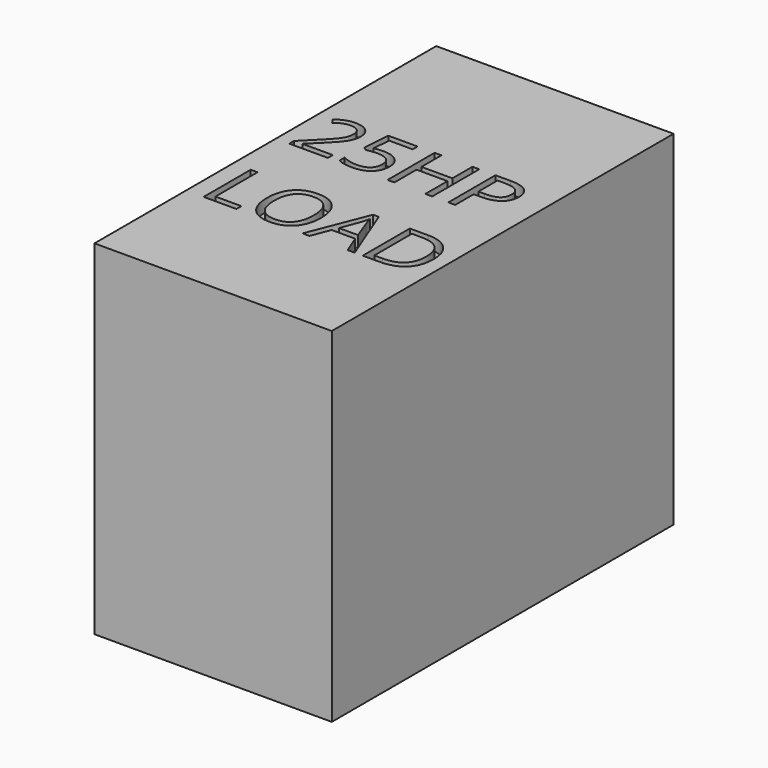
from build123d import *

# Parameters (mm, degrees)
F0_W         = 101.6
F0_H         = 182.88
F1_DEPTH     = 147.32
F2_TEXT_SIZE = 35.2777777778
F3_DEPTH     = 5


# Not quite as in the source:
# - Text() gives the source's letters only with a copy of the font that has no kerning and outlines rounded to 1/6400 em; it was checked with that copy


with BuildPart() as f1:
    # F0 (on Top) → F1 (new body)
    with BuildSketch(Plane.XY):
        Rectangle(F0_W, F0_H)
    extrude(amount=F1_DEPTH)

    # F2 (on face) → F3 (cut)
    with BuildSketch(Plane.XY.offset(147.32)):
        with Locations((-46.7696871553, 5.6050281306)):
            Text('25HP', F2_TEXT_SIZE, font='Open Sans', text_align=(TextAlign.LEFT, TextAlign.BOTTOM))
        with Locations((-46.7696871553, -42.3727496472)):
            Text('LOAD', F2_TEXT_SIZE, font='Open Sans', text_align=(TextAlign.LEFT, TextAlign.BOTTOM))
    extrude(amount=-F3_DEPTH, mode=Mode.SUBTRACT)


solid = f1.part
